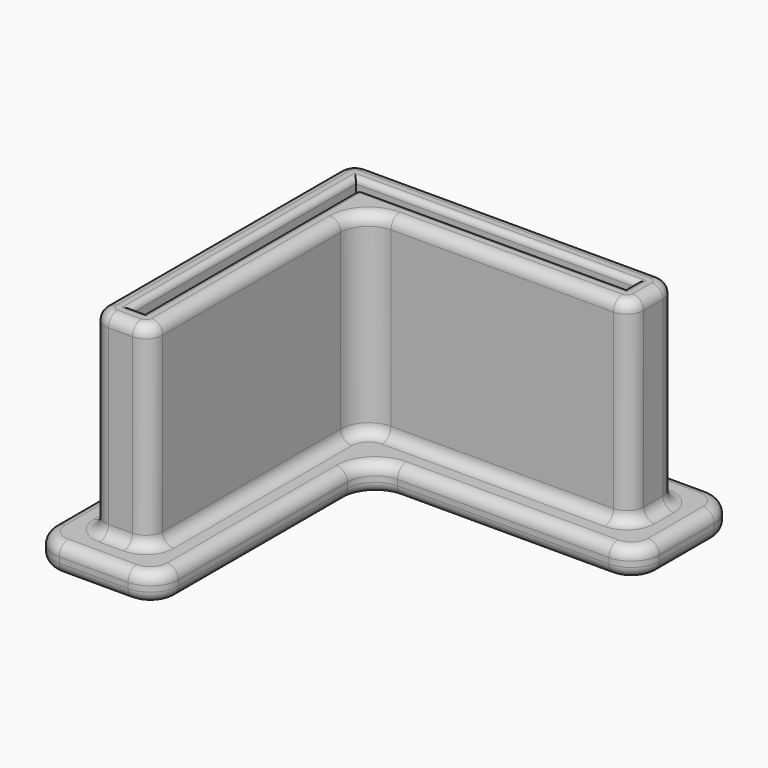
from build123d import *

# Parameters (mm, degrees)
F1_DEPTH    = 5
F2_DEPTH    = 40
F3_R        = 2
F4_R        = 1
F5_T1_DEPTH = 34
F5_S5_W     = 1
F5_S5_H     = 1
F5_T6_DEPTH = 1


# Not quite as in the source:
# - a fillet or chamfer that OpenCascade refuses, or shapes differently, is made with other operations: its cross-section is extruded or revolved along the edge and cut away or added


with BuildPart() as f1:
    # F0 (on Top) → F1 (new body)
    with BuildSketch(Plane.XY):
        Polygon((50.2, 0), (0, 0), (0, -50.2), (2.3, -50.2), (2.3, -2.3), (50.2, -2.3), align=None)
    extrude(amount=F1_DEPTH)



with BuildPart() as f1b:
    # F0 (on Top) → F1, piece 2 (new body)
    with BuildSketch(Plane.XY):
        with BuildLine():
            Line((55.2, 10), (-5, 10))
            ThreePointArc((-5, 10), (-8.5355339059, 8.5355339059), (-10, 5))
            Line((-10, 5), (-10, -55.2))
            ThreePointArc((-10, -55.2), (-8.5355339059, -58.7355339059), (-5, -60.2))
            Line((-5, -60.2), (7.3, -60.2))
            ThreePointArc((7.3, -60.2), (10.8355339059, -58.7355339059), (12.3, -55.2))
            Line((12.3, -55.2), (12.3, -17.3))
            ThreePointArc((12.3, -17.3), (13.7644660941, -13.7644660941), (17.3, -12.3))
            Line((17.3, -12.3), (55.2, -12.3))
            ThreePointArc((55.2, -12.3), (58.7355339059, -10.8355339059), (60.2, -7.3))
            Line((60.2, -7.3), (60.2, 5))
            ThreePointArc((60.2, 5), (58.7355339059, 8.5355339059), (55.2, 10))
        make_face()
        with BuildLine():
            ThreePointArc((51.2, 4), (53.3213203436, 3.1213203436), (54.2, 1))
            Line((54.2, 1), (54.2, -3.3))
            ThreePointArc((54.2, -3.3), (53.3213203436, -5.4213203436), (51.2, -6.3))
            Line((51.2, -6.3), (11.3, -6.3))
            ThreePointArc((11.3, -6.3), (7.7644660941, -7.7644660941), (6.3, -11.3))
            Line((6.3, -11.3), (6.3, -51.2))
            ThreePointArc((6.3, -51.2), (5.4213203436, -53.3213203436), (3.3, -54.2))
            Line((3.3, -54.2), (-1, -54.2))
            ThreePointArc((-1, -54.2), (-3.1213203436, -53.3213203436), (-4, -51.2))
            Line((-4, -51.2), (-4, 1))
            ThreePointArc((-4, 1), (-3.1213203436, 3.1213203436), (-1, 4))
            Line((-1, 4), (51.2, 4))
        make_face(mode=Mode.SUBTRACT)
    extrude(amount=F1_DEPTH)


with BuildPart() as f1_1:
    add(f1.part)

    add(f1b.part)  # F2 merges F1b
    # F0 (on Top) → F2 (join)
    with BuildSketch(Plane.XY):
        with BuildLine():
            Line((54.2, -3.3), (54.2, 1))
            ThreePointArc((54.2, 1), (53.3213203436, 3.1213203436), (51.2, 4))
            Line((51.2, 4), (-1, 4))
            ThreePointArc((-1, 4), (-3.1213203436, 3.1213203436), (-4, 1))
            Line((-4, 1), (-4, -51.2))
            ThreePointArc((-4, -51.2), (-3.1213203436, -53.3213203436), (-1, -54.2))
            Line((-1, -54.2), (3.3, -54.2))
            ThreePointArc((3.3, -54.2), (5.4213203436, -53.3213203436), (6.3, -51.2))
            Line((6.3, -51.2), (6.3, -11.3))
            ThreePointArc((6.3, -11.3), (7.7644660941, -7.7644660941), (11.3, -6.3))
            Line((11.3, -6.3), (51.2, -6.3))
            ThreePointArc((51.2, -6.3), (53.3213203436, -5.4213203436), (54.2, -3.3))
        make_face()
        Polygon((0, -50.2), (0, 0), (50.2, 0), (50.2, -2.3), (2.3, -2.3), (2.3, -50.2), align=None, mode=Mode.SUBTRACT)
    extrude(amount=F2_DEPTH)

    # F3
    f3_edges = [f1_1.edges().sort_by_distance(p)[0] for p in [
        (-4, -25.1, 5),
        (-10, -25.1, 5),
        (-10, -25.1, 0),
        (6.3, -31.25, 40),
        (36.25, -12.3, 0),
        (36.25, -12.3, 5),
        (13.764466, -13.764466, 0),
        (13.764466, -13.764466, 5),
        (58.735534, -10.835534, 0),
        (58.735534, -10.835534, 5),
        (60.2, -1.15, 0),
        (58.735534, 8.535534, 0),
        (25.1, 10, 0),
        (-8.535534, 8.535534, 0),
        (-8.535534, -58.735534, 0),
        (1.15, -60.2, 0),
        (10.835534, -58.735534, 0),
        (12.3, -36.25, 0),
        (60.2, -1.15, 5),
        (58.735534, 8.535534, 5),
        (25.1, 10, 5),
        (-8.535534, 8.535534, 5),
        (-8.535534, -58.735534, 5),
        (1.15, -60.2, 5),
        (10.835534, -58.735534, 5),
        (12.3, -36.25, 5),
        (53.32132, 3.12132, 5),
        (54.2, -1.15, 5),
        (53.32132, -5.42132, 5),
        (31.25, -6.3, 5),
        (7.764466, -7.764466, 5),
        (6.3, -31.25, 5),
        (5.42132, -53.32132, 5),
        (1.15, -54.2, 5),
        (-3.12132, -53.32132, 5),
        (-3.12132, 3.12132, 5),
        (25.1, 4, 5),
        (53.32132, 3.12132, 40),
        (54.2, -1.15, 40),
        (53.32132, -5.42132, 40),
        (31.25, -6.3, 40),
        (7.764466, -7.764466, 40),
        (5.42132, -53.32132, 40),
        (1.15, -54.2, 40),
        (-3.12132, -53.32132, 40),
        (-4, -25.1, 40),
        (-3.12132, 3.12132, 40),
        (25.1, 4, 40),
    ]]
    fillet(f3_edges, radius=F3_R)

    # F4
    f4_edges = [f1_1.edges().sort_by_distance(p)[0] for p in [
        (1.15, -50.2, 40),
        (50.2, -1.15, 40),
        (26.25, -2.3, 40),
        (2.3, -26.25, 40),
        (0, -25.1, 40),
        (25.1, 0, 40),
    ]]
    fillet(f4_edges, radius=F4_R)

    # F5: fillet of radius 1 on 1 edges, made by hand

    # F5_s2 → F5_t1 (cut)
    with BuildSketch(Plane.XY.offset(5)):
        with BuildLine():
            ThreePointArc((2.3, -3.3), (2.5928932188, -2.5928932188), (3.3, -2.3))
            Line((3.3, -2.3), (2.3, -2.3))
            Line((2.3, -2.3), (2.3, -3.3))
        make_face()
    extrude(amount=F5_T1_DEPTH, mode=Mode.SUBTRACT)


with BuildPart() as f5_tool4:
    # F5_s5 → F5_t6 (new body)
    with BuildSketch(Plane.YZ.offset(3.3)):
        with Locations((-2.8, 39.5)):
            Rectangle(F5_S5_W, F5_S5_H)
    extrude(amount=-F5_T6_DEPTH)

    # F5_s7 → F5_t8 (revolve, cut)
    with BuildSketch(Plane(origin=(3.3, -3.3, 39), x_dir=(0, -0.7071067812, -0.7071067812), z_dir=(0, 0.7071067812, -0.7071067812))):
        with BuildLine():
            ThreePointArc((0, -1), (1, 0), (0, 1))
            Line((0, 1), (0, -1))
        make_face()
    revolve(axis=Axis((3.3, -3.3, 39), (-1, 0, 0)), mode=Mode.SUBTRACT)


with BuildPart() as f1_2:
    add(f1_1.part)

    # F5_t3: cut F5_tool4
    add(f5_tool4.part, mode=Mode.SUBTRACT)


solid = f1_2.part
